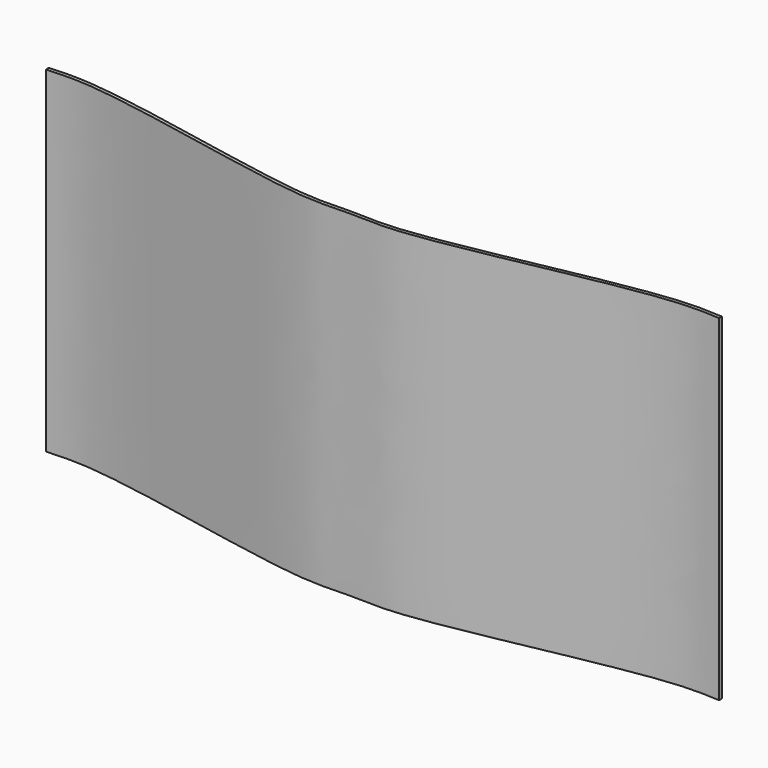
from build123d import *

# Parameters (mm, degrees)
F1_DEPTH = 1219.2


# Not quite as in the source:
# - the dataset's text gives a spline's control points without its knots; the knots are read off the source's solid


with BuildPart() as f1:
    # F0 (on Top) → F1 (new body)
    with BuildSketch(Plane.XY):
        with BuildLine():
            add(Edge.make_bspline(
                [(1219.2, 0), (1174.9872090061, 0), (1054.0337942814, -12.1344240115), (609.5779082557, 76.9354023129), (165.2357244207, 162.2202466561), (44.1330656837, 155.0539406229), (0, 152.4)],
                knots=[0, 0, 0, 0, 0.1822186894, 0.5, 0.8177813106, 1, 1, 1, 1], degree=3))
            add(Edge.make_bspline(
                [(1219.2, 0), (1263.4127909939, 0), (1384.3662057186, -12.1344240115), (1828.8220917443, 76.9354023129), (2273.1642755793, 162.2202466561), (2394.2669343163, 155.0539406229), (2438.4, 152.4)],
                knots=[0, 0, 0, 0, 0.1822186894, 0.5, 0.8177813106, 1, 1, 1, 1], degree=3))
            Line((2438.4, 152.4), (2439.1623369879, 165.0770991286))
            add(Edge.make_bspline(
                [(1219.2, 12.7), (1226.9276035352, 12.7), (1242.2994063087, 12.4351775129), (1265.700488966, 11.6631055196), (1290.0763465858, 10.9216070154), (1316.0839199325, 10.6038170736), (1339.673030638, 11.0176132238), (1360.0265559411, 11.9510281435), (1376.1148322728, 13.0059938917), (1393.1192011561, 14.4484892729), (1416.9303556227, 16.8544412679), (1448.7142553038, 20.723786661), (1489.7071734526, 26.5898185389), (1547.6803306997, 35.8328322677), (1625.4626690736, 49.6580359728), (1724.4694033709, 68.6191047427), (1826.3441813187, 88.688566061), (1928.2853645701, 108.6014590555), (2010.9723341092, 124.1797531517), (2074.3886342424, 135.5041747459), (2120.2418448295, 143.2961055187), (2164.0459538784, 150.2544428185), (2198.5609619072, 155.2481320387), (2224.814185959, 158.6937537159), (2243.7840777873, 160.9866322626), (2261.9940226456, 162.9713360414), (2276.5028265766, 164.3544906104), (2287.6920152638, 165.2895381867), (2298.5919323962, 166.1086820922), (2311.6994294694, 166.9258079001), (2326.6725552513, 167.6043703626), (2345.7249909138, 168.1460186981), (2368.0093882581, 168.2164673862), (2392.8656627405, 167.571904937), (2416.4006360579, 166.4435376989), (2431.5922528592, 165.5323259178), (2439.1623369879, 165.0770991286)],
                knots=[0, 0, 0, 0, 0.03125, 0.0625, 0.09375, 0.125, 0.15625, 0.171875, 0.1875, 0.203125, 0.21875, 0.25, 0.28125, 0.3125, 0.375, 0.4375, 0.5, 0.5625, 0.625, 0.65625, 0.6875, 0.71875, 0.75, 0.765625, 0.78125, 0.796875, 0.8125, 0.8203125, 0.828125, 0.84375, 0.859375, 0.875, 0.90625, 0.9375, 0.96875, 1, 1, 1, 1], degree=3))
            add(Edge.make_bspline(
                [(1219.2, 12.7), (1211.4723964648, 12.7), (1196.1005936913, 12.4351775129), (1172.699511034, 11.6631055196), (1148.3236534142, 10.9216070154), (1122.3160800675, 10.6038170736), (1098.726969362, 11.0176132238), (1078.3734440589, 11.9510281435), (1062.2851677272, 13.0059938917), (1045.2807988439, 14.4484892729), (1021.4696443773, 16.8544412679), (989.6857446962, 20.723786661), (948.6928265474, 26.5898185389), (890.7196693003, 35.8328322677), (812.9373309264, 49.6580359728), (713.9305966291, 68.6191047427), (612.0558186813, 88.688566061), (510.1146354299, 108.6014590555), (427.4276658908, 124.1797531517), (364.0113657576, 135.5041747459), (318.1581551705, 143.2961055187), (274.3540461216, 150.2544428185), (239.8390380928, 155.2481320387), (213.585814041, 158.6937537159), (194.6159222127, 160.9866322626), (176.4059773544, 162.9713360414), (161.8971734234, 164.3544906104), (150.7079847362, 165.2895381867), (139.8080676038, 166.1086820922), (126.7005705306, 166.9258079001), (111.7274447487, 167.6043703626), (92.6750090862, 168.1460186981), (70.3906117419, 168.2164673862), (45.5343372595, 167.571904937), (21.9993639421, 166.4435376989), (6.8077471408, 165.5323259178), (-0.7623369879, 165.0770991286)],
                knots=[0, 0, 0, 0, 0.03125, 0.0625, 0.09375, 0.125, 0.15625, 0.171875, 0.1875, 0.203125, 0.21875, 0.25, 0.28125, 0.3125, 0.375, 0.4375, 0.5, 0.5625, 0.625, 0.65625, 0.6875, 0.71875, 0.75, 0.765625, 0.78125, 0.796875, 0.8125, 0.8203125, 0.828125, 0.84375, 0.859375, 0.875, 0.90625, 0.9375, 0.96875, 1, 1, 1, 1], degree=3))
            Line((-0.7623369879, 165.0770991286), (0, 152.4))
        make_face()
    extrude(amount=F1_DEPTH)


solid = f1.part
